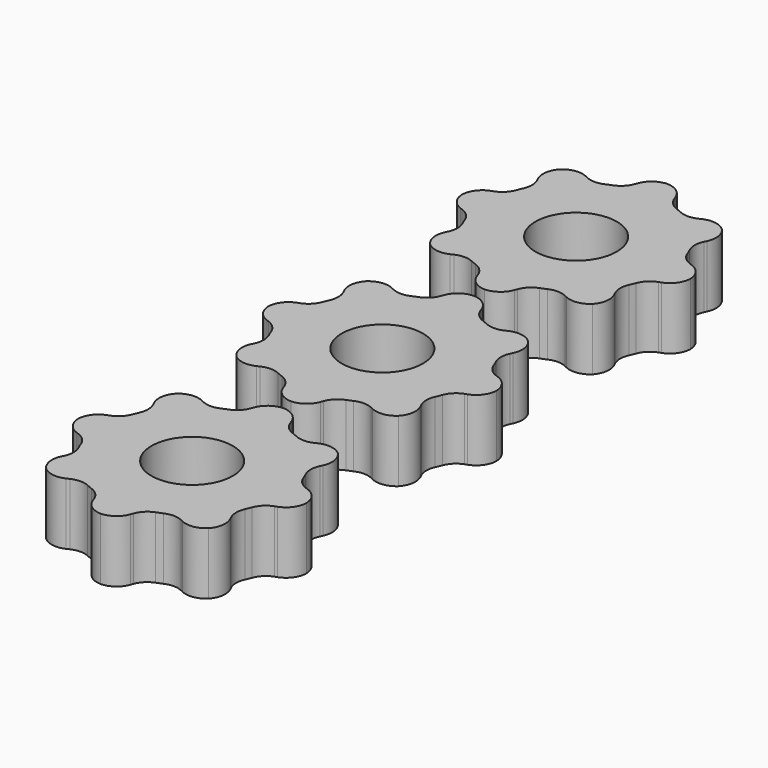
from build123d import *

# Parameters (mm, degrees)
F0_R        = 2.985970541
F1_DEPTH    = 4.5511212
F2_DEPTH    = 4.5511212
F3_T1_DEPTH = 4.5511212
F3_T3_DEPTH = 9.9145633344
F3_T5_DEPTH = 9.9145633387


# Not quite as in the source:
# - a fillet or chamfer that OpenCascade refuses, or shapes differently, is made with other operations: its cross-section is extruded or revolved along the edge and cut away or added


with BuildPart() as f1:
    # F0 (on Top) → F1 (new body)
    with BuildSketch(Plane.XY):
        with BuildLine():
            ThreePointArc((-7.7955871708, 60.0406383768), (-7.6315265379, 60.8840448824), (-7.5765393856, 61.7414985768))
            ThreePointArc((-7.5765393856, 61.7414985768), (-7.6315265379, 62.5989522713), (-7.7955871708, 63.4423587768))
            ThreePointArc((-7.7955871708, 63.4423587768), (-8.0875311817, 64.3104278137), (-8.4949130944, 65.1306809061))
            ThreePointArc((-8.4949130944, 65.1306809061), (-9.5427127013, 66.4882608617), (-10.900292657, 67.5360604686))
            ThreePointArc((-10.900292657, 67.5360604686), (-11.720545656, 67.9434423427), (-12.5886145908, 68.235386341))
            ThreePointArc((-12.5886145908, 68.235386341), (-14.2894749862, 68.4544341775), (-15.9903353816, 68.235386341))
            ThreePointArc((-15.9903353816, 68.235386341), (-16.8584043164, 67.9434423427), (-17.6786573154, 67.5360604686))
            ThreePointArc((-17.6786573154, 67.5360604686), (-19.0362372711, 66.4882608617), (-20.084036878, 65.1306809061))
            ThreePointArc((-20.084036878, 65.1306809061), (-20.4914187907, 64.3104278137), (-20.7833628016, 63.4423587768))
            ThreePointArc((-20.7833628016, 63.4423587768), (-21.0024105868, 61.7414985768), (-20.7833628016, 60.0406383768))
            ThreePointArc((-20.7833628016, 60.0406383768), (-20.4914191182, 59.1725701306), (-20.0840377422, 58.3523177251))
            ThreePointArc((-20.0840377422, 58.3523177251), (-19.0362384814, 56.9947375023), (-17.6786587929, 55.9469375492))
            ThreePointArc((-17.6786587929, 55.9469375492), (-16.8584050138, 55.5395550999), (-15.9903351862, 55.2476107615))
            ThreePointArc((-15.9903351862, 55.2476107615), (-14.2894749862, 55.0285629762), (-12.5886147862, 55.2476107615))
            ThreePointArc((-12.5886147862, 55.2476107615), (-11.72054654, 55.5395544448), (-10.9002941345, 55.9469358209))
            ThreePointArc((-10.9002941345, 55.9469358209), (-9.5427139116, 56.9947350816), (-8.4949139586, 58.3523147701))
            ThreePointArc((-8.4949139586, 58.3523147701), (-8.0875315092, 59.1725685493), (-7.7955871708, 60.0406383768))
        make_face()
        with Locations((-14.2894749862, 61.7414985768)):
            Circle(F0_R, mode=Mode.SUBTRACT)
    extrude(amount=F1_DEPTH)

    # F0 (on Top) → F2 (join)
    with BuildSketch(Plane.XY):
        with BuildLine():
            ThreePointArc((-20.7833628016, 60.0406383768), (-21.0024105868, 61.7414985768), (-20.7833628016, 63.4423587768))
            Line((-20.7833628016, 63.4423587768), (-22.6607766938, 62.769432043))
            Line((-22.6607766938, 62.769432043), (-22.6607766938, 60.7135651107))
            Line((-22.6607766938, 60.7135651107), (-20.7833628016, 60.0406383768))
        make_face()
        with BuildLine():
            ThreePointArc((-15.9903353816, 68.235386341), (-14.2894749862, 68.4544341775), (-12.5886145908, 68.235386341))
            Line((-12.5886145908, 68.235386341), (-13.2652480473, 70.1231417047))
            Line((-13.2652480473, 70.1231417047), (-15.3137019267, 70.1231417047))
            Line((-15.3137019267, 70.1231417047), (-15.9903353816, 68.235386341))
        make_face()
        with BuildLine():
            ThreePointArc((-20.084036878, 65.1306809061), (-19.0362372711, 66.4882608617), (-17.6786573154, 67.5360604686))
            Line((-17.6786573154, 67.5360604686), (-19.5154104475, 68.4035310873))
            Line((-19.5154104475, 68.4035310873), (-20.9515074966, 66.9674340382))
            Line((-20.9515074966, 66.9674340382), (-20.084036878, 65.1306809061))
        make_face()
        with BuildLine():
            ThreePointArc((-10.900292657, 67.5360604686), (-9.5427127013, 66.4882608617), (-8.4949130944, 65.1306809061))
            Line((-8.4949130944, 65.1306809061), (-7.6274424758, 66.9674340382))
            Line((-7.6274424758, 66.9674340382), (-9.0635395249, 68.4035310873))
            Line((-9.0635395249, 68.4035310873), (-10.900292657, 67.5360604686))
        make_face()
        with BuildLine():
            ThreePointArc((-7.7955871708, 63.4423587768), (-7.6315265379, 62.5989522713), (-7.5765393856, 61.7414985768))
            ThreePointArc((-7.5765393856, 61.7414985768), (-7.6315265379, 60.8840448824), (-7.7955871708, 60.0406383768))
            Line((-7.7955871708, 60.0406383768), (-5.9089133301, 60.71688418))
            Line((-5.9089133301, 60.71688418), (-5.9089133301, 62.7661129737))
            Line((-5.9089133301, 62.7661129737), (-7.7955871708, 63.4423587768))
        make_face()
        with BuildLine():
            Line((-7.6266341219, 56.513847013), (-8.4949139586, 58.3523147701))
            ThreePointArc((-8.4949139586, 58.3523147701), (-9.5427139116, 56.9947350816), (-10.9002941345, 55.9469358209))
            Line((-10.9002941345, 55.9469358209), (-9.0618268202, 55.0786550467))
            Line((-9.0618268202, 55.0786550467), (-7.6266341219, 56.513847013))
        make_face()
        with BuildLine():
            Line((-13.2683575849, 53.3511805719), (-12.5886147862, 55.2476107615))
            ThreePointArc((-12.5886147862, 55.2476107615), (-14.2894749862, 55.0285629762), (-15.9903351862, 55.2476107615))
            Line((-15.9903351862, 55.2476107615), (-15.3105923875, 53.3511805719))
            Line((-15.3105923875, 53.3511805719), (-13.2683575849, 53.3511805719))
        make_face()
        with BuildLine():
            Line((-19.5308540518, 55.0721744262), (-17.6786587929, 55.9469375492))
            ThreePointArc((-17.6786587929, 55.9469375492), (-19.0362384814, 56.9947375023), (-20.0840377422, 58.3523177251))
            Line((-20.0840377422, 58.3523177251), (-20.9588018098, 56.5001229123))
            Line((-20.9588018098, 56.5001229123), (-19.5308540518, 55.0721744262))
        make_face()
    extrude(amount=F2_DEPTH)

    # F3: fillet of radius 1.524 on 32 edges, made by hand

    # F3_s2 → F3_t1 (join)
    with BuildSketch(Plane.XY):
        with BuildLine():
            ThreePointArc((-11.9410325911, 68.030244294), (-12.4926151246, 68.3874647422), (-12.8425064995, 68.9437252618))
            Line((-12.8425064995, 68.9437252618), (-12.5886145908, 68.235386341))
            ThreePointArc((-12.5886145908, 68.235386341), (-12.2622270766, 68.1410118624), (-11.9410325911, 68.030244294))
        make_face()
        with BuildLine():
            ThreePointArc((-11.5032596254, 67.8489127876), (-10.8606388577, 67.7114780222), (-10.2198926882, 67.857403044))
            Line((-10.2198926882, 67.857403044), (-10.900292657, 67.5360604686))
            ThreePointArc((-10.900292657, 67.5360604686), (-11.1978163212, 67.7001184739), (-11.5032596254, 67.8489127876))
        make_face()
        with BuildLine():
            ThreePointArc((-8.1820607755, 64.5277139377), (-8.3194955409, 65.1703347053), (-8.173570519, 65.8110808748))
            Line((-8.173570519, 65.8110808748), (-8.4949130944, 65.1306809061))
            ThreePointArc((-8.4949130944, 65.1306809061), (-8.3308550892, 64.8331572419), (-8.1820607755, 64.5277139377))
        make_face()
        with BuildLine():
            ThreePointArc((-8.0007292068, 64.0899408053), (-7.6435087589, 63.5383582482), (-7.0872482249, 63.1884668592))
            Line((-7.0872482249, 63.1884668592), (-7.7955871708, 63.4423587768))
            ThreePointArc((-7.7955871708, 63.4423587768), (-7.8899616433, 63.7687463054), (-8.0007292068, 64.0899408053))
        make_face()
        with BuildLine():
            ThreePointArc((-8.0007292068, 59.3930563484), (-7.6435087589, 59.9446389055), (-7.0872482249, 60.2945302945))
            Line((-7.0872482249, 60.2945302945), (-7.7955871708, 60.0406383768))
            ThreePointArc((-7.7955871708, 60.0406383768), (-7.8899616433, 59.7142508483), (-8.0007292068, 59.3930563484))
        make_face()
        with BuildLine():
            ThreePointArc((-8.1820614859, 58.9552816588), (-8.3194964152, 58.3126609262), (-8.1735715567, 57.6719147194))
            Line((-8.1735715567, 57.6719147194), (-8.4949139586, 58.3523147701))
            ThreePointArc((-8.4949139586, 58.3523147701), (-8.3308558775, 58.6498383925), (-8.1820614859, 58.9552816588))
        make_face()
        with BuildLine():
            ThreePointArc((-11.5032611827, 55.6340836557), (-10.86064038, 55.7715182573), (-10.2198942477, 55.625593072))
            Line((-10.2198942477, 55.625593072), (-10.9002941345, 55.9469358209))
            ThreePointArc((-10.9002941345, 55.9469358209), (-11.1978178405, 55.7828778915), (-11.5032611827, 55.6340836557))
        make_face()
        with BuildLine():
            ThreePointArc((-11.9410327577, 55.4527527974), (-12.4926153149, 55.0955323495), (-12.8425067039, 54.5392718155))
            Line((-12.8425067039, 54.5392718155), (-12.5886147862, 55.2476107615))
            ThreePointArc((-12.5886147862, 55.2476107615), (-12.2622272576, 55.341985234), (-11.9410327577, 55.4527527974))
        make_face()
        with BuildLine():
            ThreePointArc((-16.6379172147, 55.4527527974), (-16.0863346575, 55.0955323495), (-15.7364432685, 54.5392718155))
            Line((-15.7364432685, 54.5392718155), (-15.9903351862, 55.2476107615))
            ThreePointArc((-15.9903351862, 55.2476107615), (-16.3167227148, 55.341985234), (-16.6379172147, 55.4527527974))
        make_face()
        with BuildLine():
            ThreePointArc((-17.0756919043, 55.6340850765), (-17.7183126369, 55.7715200058), (-18.3590588436, 55.6255951473))
            Line((-18.3590588436, 55.6255951473), (-17.6786587929, 55.9469375492))
            ThreePointArc((-17.6786587929, 55.9469375492), (-17.3811351705, 55.7828794681), (-17.0756919043, 55.6340850765))
        make_face()
        with BuildLine():
            ThreePointArc((-20.5782207656, 59.3930563484), (-20.9354412135, 59.9446389055), (-21.4917017475, 60.2945302945))
            Line((-21.4917017475, 60.2945302945), (-20.7833628016, 60.0406383768))
            ThreePointArc((-20.7833628016, 60.0406383768), (-20.6889883291, 59.7142508483), (-20.5782207656, 59.3930563484))
        make_face()
        with BuildLine():
            ThreePointArc((-20.3968899074, 58.9552847733), (-20.2594553058, 58.3126639706), (-20.405380491, 57.6719178383))
            Line((-20.405380491, 57.6719178383), (-20.0840377422, 58.3523177251))
            ThreePointArc((-20.0840377422, 58.3523177251), (-20.2480956716, 58.6498414312), (-20.3968899074, 58.9552847733))
        make_face()
        with BuildLine():
            ThreePointArc((-20.5782207656, 64.0899408053), (-20.9354412135, 63.5383582482), (-21.4917017475, 63.1884668592))
            Line((-21.4917017475, 63.1884668592), (-20.7833628016, 63.4423587768))
            ThreePointArc((-20.7833628016, 63.4423587768), (-20.6889883291, 63.7687463054), (-20.5782207656, 64.0899408053))
        make_face()
        with BuildLine():
            ThreePointArc((-17.075690347, 67.8489127876), (-17.7183111147, 67.7114780222), (-18.3590572842, 67.857403044))
            Line((-18.3590572842, 67.857403044), (-17.6786573154, 67.5360604686))
            ThreePointArc((-17.6786573154, 67.5360604686), (-17.3811336512, 67.7001184739), (-17.075690347, 67.8489127876))
        make_face()
        with BuildLine():
            ThreePointArc((-16.6379173818, 68.0302442938), (-16.086334848, 68.3874647424), (-15.7364434733, 68.9437252627))
            Line((-15.7364434733, 68.9437252627), (-15.9903353816, 68.235386341))
            ThreePointArc((-15.9903353816, 68.235386341), (-16.3167228961, 68.1410118623), (-16.6379173818, 68.0302442938))
        make_face()
        with BuildLine():
            ThreePointArc((-20.3968891969, 64.5277139377), (-20.2594544315, 65.1703347053), (-20.4053794534, 65.8110808748))
            Line((-20.4053794534, 65.8110808748), (-20.084036878, 65.1306809061))
            ThreePointArc((-20.084036878, 65.1306809061), (-20.2480948832, 64.8331572419), (-20.3968891969, 64.5277139377))
        make_face()
    extrude(amount=F3_T1_DEPTH)

    # F3_s4 → F3_t3 (cut)
    with BuildSketch(Plane.XY.offset(-2.6817210672)):
        with BuildLine():
            ThreePointArc((-5.9089133301, 61.6934245468), (-6.1866702546, 62.5706099301), (-6.9186957405, 63.1280521188))
            Line((-6.9186957405, 63.1280521188), (-5.9089133301, 62.7661129737))
            Line((-5.9089133301, 62.7661129737), (-5.9089133301, 61.6934245468))
        make_face()
        with BuildLine():
            ThreePointArc((-6.9186957405, 60.3549450349), (-6.1866702546, 60.9123872236), (-5.9089133301, 61.7895726069))
            Line((-5.9089133301, 61.7895726069), (-5.9089133301, 60.71688418))
            Line((-5.9089133301, 60.71688418), (-6.9186957405, 60.3549450349))
        make_face()
        with BuildLine():
            ThreePointArc((-8.3851395761, 55.7553419457), (-7.9612794398, 56.5720093754), (-8.0847282406, 57.4838007437))
            Line((-8.0847282406, 57.4838007437), (-7.6266341219, 56.513847013))
            Line((-7.6266341219, 56.513847013), (-8.3851395761, 55.7553419457))
        make_face()
        with BuildLine():
            ThreePointArc((-10.0317803172, 55.53674966), (-9.1199890118, 55.4133003942), (-8.303321366, 55.837160114))
            Line((-8.303321366, 55.837160114), (-9.0618268202, 55.0786550467))
            Line((-9.0618268202, 55.0786550467), (-10.0317803172, 55.53674966))
        make_face()
        with BuildLine():
            ThreePointArc((-14.3410460118, 53.3511805719), (-13.4638606285, 53.6289374963), (-12.9064184397, 54.3609629823))
            Line((-12.9064184397, 54.3609629823), (-13.2683575849, 53.3511805719))
            Line((-13.2683575849, 53.3511805719), (-14.3410460118, 53.3511805719))
        make_face()
        with BuildLine():
            ThreePointArc((-15.6725315327, 54.3609629823), (-15.1150893439, 53.6289374963), (-14.2379039606, 53.3511805719))
            Line((-14.2379039606, 53.3511805719), (-15.3105923875, 53.3511805719))
            Line((-15.3105923875, 53.3511805719), (-15.6725315327, 54.3609629823))
        make_face()
        with BuildLine():
            ThreePointArc((-20.2893591192, 55.8306798803), (-19.4726916895, 55.406819744), (-18.5609003212, 55.5302685448))
            Line((-18.5609003212, 55.5302685448), (-19.5308540518, 55.0721744262))
            Line((-19.5308540518, 55.0721744262), (-20.2893591192, 55.8306798803))
        make_face()
        with BuildLine():
            ThreePointArc((-20.5007071965, 57.4700764094), (-20.6241564623, 56.558285104), (-20.2002967424, 55.7416174582))
            Line((-20.2002967424, 55.7416174582), (-20.9588018098, 56.5001229123))
            Line((-20.9588018098, 56.5001229123), (-20.5007071965, 57.4700764094))
        make_face()
        with BuildLine():
            ThreePointArc((-22.6607766938, 61.7862535376), (-22.3830197693, 60.9090681542), (-21.6509942834, 60.3516259655))
            Line((-21.6509942834, 60.3516259655), (-22.6607766938, 60.7135651107))
            Line((-22.6607766938, 60.7135651107), (-22.6607766938, 61.7862535376))
        make_face()
        with BuildLine():
            ThreePointArc((-21.6509942834, 63.1313711882), (-22.3830197693, 62.5739289995), (-22.6607766938, 61.6967436161))
            Line((-22.6607766938, 61.6967436161), (-22.6607766938, 62.769432043))
            Line((-22.6607766938, 62.769432043), (-21.6509942834, 63.1313711882))
        make_face()
        with BuildLine():
            ThreePointArc((-20.1930022359, 67.7259392989), (-20.616862164, 66.9092717612), (-20.4934131307, 65.9974804243))
            Line((-20.4934131307, 65.9974804243), (-20.9515074966, 66.9674340382))
            Line((-20.9515074966, 66.9674340382), (-20.1930022359, 67.7259392989))
        make_face()
        with BuildLine():
            ThreePointArc((-18.5454568337, 67.9454367213), (-19.4572481705, 68.0688857546), (-20.2739157083, 67.6450258265))
            Line((-20.2739157083, 67.6450258265), (-19.5154104475, 68.4035310873))
            Line((-19.5154104475, 68.4035310873), (-18.5454568337, 67.9454367213))
        make_face()
        with BuildLine():
            ThreePointArc((-12.9033089021, 69.1133592943), (-13.4607510909, 69.8453847802), (-14.3379364742, 70.1231417047))
            Line((-14.3379364742, 70.1231417047), (-13.2652480473, 70.1231417047))
            Line((-13.2652480473, 70.1231417047), (-12.9033089021, 69.1133592943))
        make_face()
        with BuildLine():
            ThreePointArc((-8.3050342641, 67.6450258265), (-9.1217018019, 68.0688857546), (-10.0334931387, 67.9454367213))
            Line((-10.0334931387, 67.9454367213), (-9.0635395249, 68.4035310873))
            Line((-9.0635395249, 68.4035310873), (-8.3050342641, 67.6450258265))
        make_face()
        with BuildLine():
            ThreePointArc((-8.0855368417, 65.9974804243), (-7.9620878084, 66.9092717612), (-8.3859477365, 67.7259392989))
            Line((-8.3859477365, 67.7259392989), (-7.6274424758, 66.9674340382))
            Line((-7.6274424758, 66.9674340382), (-8.0855368417, 65.9974804243))
        make_face()
    extrude(amount=F3_T3_DEPTH, mode=Mode.SUBTRACT)

    # F3_s6 → F3_t5 (cut)
    with BuildSketch(Plane.XY.offset(-2.6817210693)):
        with BuildLine():
            ThreePointArc((-14.241013499, 70.1231417047), (-15.1181988828, 69.8453847799), (-15.6756410714, 69.1133592932))
            Line((-15.6756410714, 69.1133592932), (-15.3137019267, 70.1231417047))
            Line((-15.3137019267, 70.1231417047), (-14.241013499, 70.1231417047))
        make_face()
    extrude(amount=F3_T5_DEPTH, mode=Mode.SUBTRACT)


with BuildPart() as f4_1:
    # F4: copy of F1
    add(f1.part.moved(Location((0, -17.78, 0))))


with BuildPart() as f5_1:
    # F5: copy of F4_1
    add(f4_1.part.moved(Location((0.2032, -17.7038, 0))))


solid = Compound([f1.part, f4_1.part, f5_1.part])
